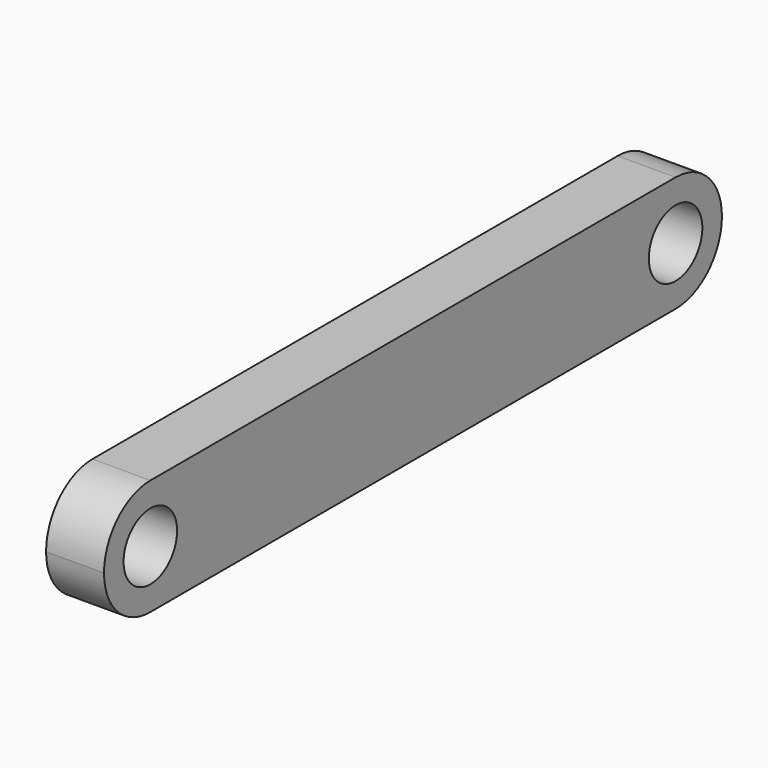
from build123d import *

# Parameters (mm, degrees)
F0_W     = 19.05
F0_H     = 38.1
F1_DEPTH = 254
F3_D     = 22
F4_R     = 19.04999
F5_R     = 1.190625
F6_DEPTH = 12.7


# Not quite as in the source:
# - a fillet or chamfer is up to 0.001 mm smaller than in the source, because OpenCascade refuses the exact size


with BuildPart() as f1:
    # F0 (on Front) → F1 (new body)
    with BuildSketch(Plane.XZ):
        Rectangle(F0_W, F0_H)
    extrude(amount=-F1_DEPTH)

    # F3 (through all)
    with Locations(Plane.YZ.offset(9.525)):
        with Locations((19.05, 0), (234.95, 0)):
            Hole(F3_D / 2)

    # F4 (radius 19.05 in the source; OpenCascade refuses exactly that, so slightly less here)
    f4_edges = [f1.edges().sort_by_distance(p)[0] for p in [
        (0, 0, 19.05),
        (0, 0, -19.05),
        (0, 254, 19.05),
        (0, 254, -19.05),
    ]]
    fillet(f4_edges, radius=F4_R)

    # F5 (on face) → F6 (cut)
    with BuildSketch(Plane(origin=(0, 0, -19.05), x_dir=(1, 0, 0), z_dir=(0, 0, -1))):
        with Locations((0, -103.98125)):
            Circle(F5_R)
        with Locations((0, -69.85)):
            Circle(F5_R)
    extrude(amount=-F6_DEPTH, mode=Mode.SUBTRACT)


solid = f1.part
